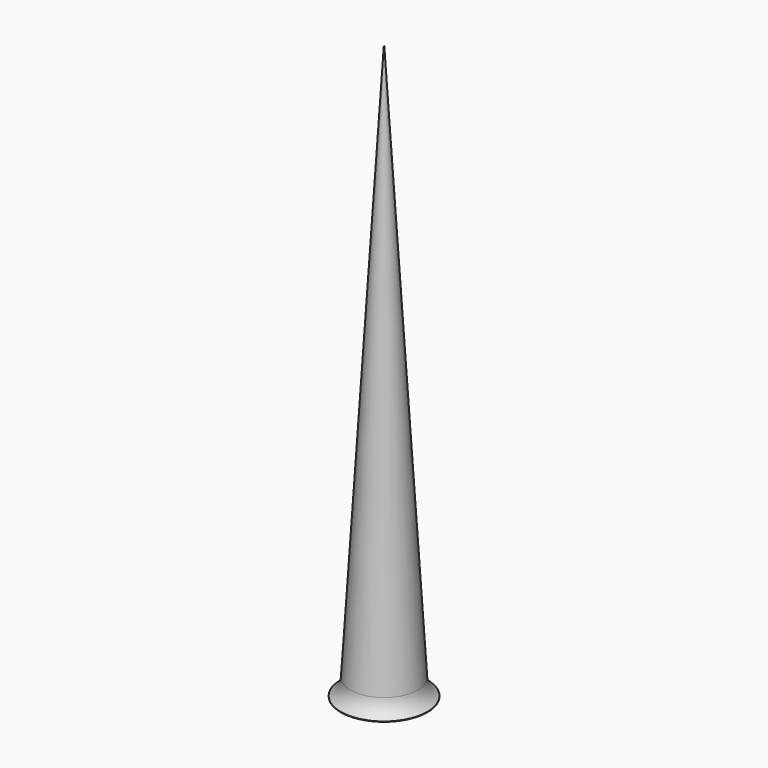
from build123d import *

# Parameters (mm, degrees)
F0_R     = 85
F2_R     = 0.5
F4_R     = 105.9677495378
F5_DEPTH = 1


# Not quite as in the source:
# - a fillet or chamfer that OpenCascade refuses, or shapes differently, is made with other operations: its cross-section is extruded or revolved along the edge and cut away or added


with BuildPart() as f3:
    # F0 (on Top) → F3 section 0
    with BuildSketch(Plane.XY):
        Circle(F0_R)
    # F2 (on offset) → F3 section 1
    with BuildSketch(Plane.XY.offset(1400)):
        Circle(F2_R)
    loft()

    # F4 (on Top) → F5 (join)
    with BuildSketch(Plane.XY):
        Circle(F4_R)
    extrude(amount=F5_DEPTH)

    # F6: fillet of radius 50 on 1 edges, made by hand


with BuildPart() as f6_tool2:
    # F6_s3 → F6_t4 (revolve)
    with BuildSketch(Plane.XZ):
        with BuildLine():
            ThreePointArc((105.9675375029, 0.9996608228), (89.4883112296, 17.8541588617), (82.5620399387, 40.3855984233))
            Line((82.5620399387, 40.3855984233), (77.5709757484, 40.0843520489))
            ThreePointArc((77.5709757484, 40.0843520489), (78.7599768444, 20.3915648868), (79.9485786669, 0.6987536257))
            Line((79.9485786669, 0.6987536257), (84.9396428571, -4.0001471107))
            ThreePointArc((84.9396428571, -4.0001471107), (95.45359018, -4.0001471107), (103.3170230691, -3.2401793116))
            Line((103.3170230691, -3.2401793116), (105.9675375029, 0.9996608228))
        make_face()
    revolve(axis=Axis((0, 0, 1), (0, 0, 1)))

    split(bisect_by=Plane.XY, keep=Keep.TOP)


with BuildPart() as f3_1:
    add(f3.part)

    # F6_t1: union F6_tool2
    add(f6_tool2.part)


solid = f3_1.part
